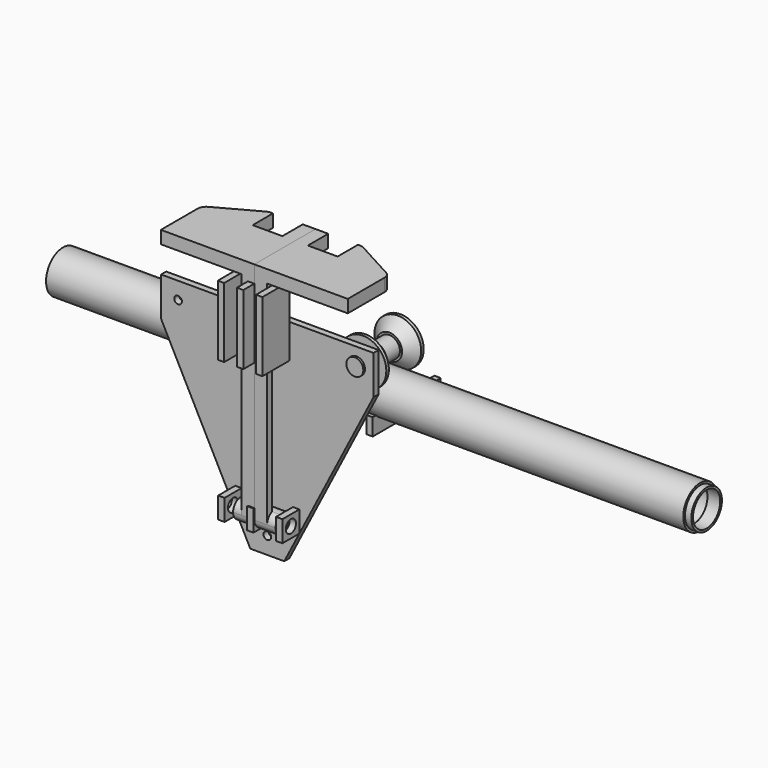
from build123d import *

# Parameters (mm, degrees)
F0_R      = 50
F0_R_2    = 45
F1_DEPTH  = 750
F2_W      = 35
F2_H      = 2.5
F6_SIZE   = 0.5
F8_DEPTH  = 15
F9_R      = 15.5
F9_R_2    = 12
F9_R_3    = 9.5
F9_R_4    = 9
F10_DEPTH = 3
F11_R     = 9
F11_R_2   = 15.5
F12_DEPTH = 15
F16_W     = 10
F16_H     = 50
F17_DEPTH = 50
F18_R     = 50
F19_DEPTH = 545.001
F21_R     = 2.5
F22_DEPTH = 12.5
F23_DEPTH = 15
F24_W     = 15
F24_H     = 50
F25_DEPTH = 50
F26_R     = 15
F27_DEPTH = 615.4994894868
F28_R     = 15
F29_DEPTH = 50
F28_W     = 15
F28_H     = 475
F30_DEPTH = 30
F31_DEPTH = 220
F32_W     = 70
F32_H     = 60
F33_DEPTH = 624.001
F34_DEPTH = 50
F35_DEPTH = 30
F36_DEPTH = 220
F37_DEPTH = 624.001
F38_R     = 45
F38_R_2   = 40
F39_DEPTH = 15
F40_W     = 15
F40_H     = 80
F40_H_2   = 84
F41_DEPTH = 80


with BuildPart() as f1:
    # F0 (on Right) → F1 (new body, symmetric)
    with BuildSketch(Plane.YZ):
        Circle(F0_R)
        Circle(F0_R_2, mode=Mode.SUBTRACT)
    extrude(amount=F1_DEPTH, both=True)

    # F38 (on face) → F39 (join, symmetric)
    with BuildSketch(Plane.YZ.offset(750)):
        Circle(F38_R)
        Circle(F38_R_2, mode=Mode.SUBTRACT)
    extrude(amount=F39_DEPTH, both=True)


with BuildPart() as f3:
    # F2 (on Right) → F3 (revolve)
    with BuildSketch(Plane.YZ):
        with Locations((0, 66.9606781187)):
            Rectangle(F2_W, F2_H)
        Polygon((-17.5, 65.7106781187), (-55, 65.7106781187), (-55, 23.2106781187), (-47.5, 23.2106781187), (-22.5, 48.2106781187), (-22.5, 53.2106781187), (22.5, 53.2106781187), (22.5, 48.2106781187), (47.5, 23.2106781187), (55, 23.2106781187), (55, 65.7106781187), (17.5, 65.7106781187), align=None)
    revolve(axis=Axis((0, 60.7904960771, 78.2106781187), (0, 1, 0)))


with BuildPart() as f5:
    # F4 (on face) → F5 (revolve)
    with BuildSketch(Plane.YZ):
        Polygon((-56, 65.7106781187), (-55, 65.7106781187), (-17.5, 65.7106781187), (-17.5, 68.2106781187), (-17.5, 69.2106781187), (-56, 69.2106781187), align=None)
    revolve(axis=Axis((0, 60.7904960771, 78.2106781187), (0, 1, 0)))

    # F6
    f6_edges = [f5.edges().sort_by_distance(p)[0] for p in [
        (0, -56, 87.210678),
        (0, -17.5, 87.210678),
        (0, -17.5, 90.710678),
        (0, -56, 90.710678),
    ]]
    chamfer(f6_edges, length=F6_SIZE)


with BuildPart() as f8:
    # F7 (on Right) → F8 (new body)
    with BuildSketch(Plane.YZ):
        with BuildLine():
            ThreePointArc((35.7071421427, -35), (0, -50), (-35.7071421427, -35))
            Line((-35.7071421427, -35), (-45, -35))
            Line((-45, -35), (-45, -75))
            Line((-45, -75), (155, -75))
            Line((155, -75), (155, -35))
            Line((155, -35), (35.7071421427, -35))
        make_face()
    extrude(amount=F8_DEPTH)


with BuildPart() as f10:
    # F9 (on face) → F10 (new body)
    with BuildSketch(Plane.XZ.offset(56)):
        with Locations((0, 78.2106781187)):
            Circle(F9_R)
        with Locations((0, 78.2106781187)):
            Circle(F9_R_2, mode=Mode.SUBTRACT)
        with Locations((0, 78.2106781187)):
            Circle(F9_R_2)
        with Locations((0, 78.2106781187)):
            Circle(F9_R_3, mode=Mode.SUBTRACT)
        with Locations((0, 78.2106781187)):
            Circle(F9_R_3)
        with Locations((0, 78.2106781187)):
            Circle(F9_R_4, mode=Mode.SUBTRACT)
    extrude(amount=F10_DEPTH)


with BuildPart() as f12:
    # F11 (on face) → F12 (new body)
    with BuildSketch(Plane.XZ.offset(59)):
        Polygon((40, 118.2106781187), (-460, 118.2106781187), (-460, 26.3970603982), (-250, -381.7893218813), (-170, -381.7893218813), (40, 26.3970603982), align=None)
        with Locations((-210, -341.7893218813)):
            Circle(F11_R, mode=Mode.SUBTRACT)
        with Locations((-420, 78.2106781187)):
            Circle(F11_R, mode=Mode.SUBTRACT)
        with Locations((-210, -78.2106781187)):
            Circle(F11_R, mode=Mode.SUBTRACT)
        with Locations((0, 78.2106781187)):
            Circle(F11_R_2, mode=Mode.SUBTRACT)
        with Locations((0, 78.2106781187)):
            Circle(F11_R_2)
        with Locations((0, 78.2106781187)):
            Circle(F11_R, mode=Mode.SUBTRACT)
    extrude(amount=F12_DEPTH)

    # F16 (on face) → F17 (join)
    with BuildSketch(Plane(origin=(0, -59, 0), x_dir=(-1, 0, 0), z_dir=(0, 1, 0))):
        with Locations((210, 0)):
            Rectangle(F16_W, F16_H)
        with Locations((210, -263.5786437627)):
            Rectangle(F16_W, F16_H)
    extrude(amount=F17_DEPTH)

    # F18 (on face) → F19 (cut, through all)
    with BuildSketch(Plane.YZ.offset(-205)):
        with Locations((0, -263.5786437627)):
            Circle(F18_R)
        with BuildLine():
            ThreePointArc((-43.3012701892, -25), (12.9409522551, -48.2962913145), (50, 0))
            ThreePointArc((50, 0), (12.9409522551, 48.2962913145), (-43.3012701892, 25))
            Line((-43.3012701892, 25), (-9, 25))
            Line((-9, 25), (-9, -25))
            Line((-9, -25), (-43.3012701892, -25))
        make_face()
        with BuildLine():
            Line((-9, 25), (-43.3012701892, 25))
            ThreePointArc((-43.3012701892, 25), (-50, 0), (-43.3012701892, -25))
            Line((-43.3012701892, -25), (-9, -25))
            Line((-9, -25), (-9, 25))
        make_face()
    extrude(amount=-F19_DEPTH, mode=Mode.SUBTRACT)

    # F24 (on face) → F25 (join)
    with BuildSketch(Plane.XZ.offset(74)):
        with Locations((-142.0015105132, -287.7893218813)):
            Rectangle(F24_W, F24_H)
        with Locations((-277.9984894868, -287.7893218813)):
            Rectangle(F24_W, F24_H)
        with Locations((-210, -287.7893218813)):
            Rectangle(F24_W, F24_H)
    extrude(amount=F25_DEPTH)

    # F26 (on face) → F27 (cut, through all)
    with BuildSketch(Plane.YZ.offset(-134.5015105132)):
        with Locations((-99, -287.7893218813)):
            Circle(F26_R)
    extrude(amount=-F27_DEPTH, mode=Mode.SUBTRACT)

    # F40 (on face) → F41 (join)
    with BuildSketch(Plane.XZ.offset(74)):
        with Locations((-255, 78.2106781187)):
            Rectangle(F40_W, F40_H)
        with Locations((-210, 78.2106781187)):
            Rectangle(F40_W, F40_H)
        with Locations((-165, 78.2106781187)):
            Rectangle(F40_W, F40_H)
        with Locations((-255, 160.2106781187)):
            Rectangle(F40_W, F40_H_2)
        with Locations((-210, 160.2106781187)):
            Rectangle(F40_W, F40_H_2)
        with Locations((-165, 160.2106781187)):
            Rectangle(F40_W, F40_H_2)
    extrude(amount=F41_DEPTH)


with BuildPart() as f15:
    # F14 (on Right) → F15 (revolve)
    with BuildSketch(Plane.YZ):
        Polygon((-74, 58.2106781187), (-74, 69.2106781187), (-74, 78.2106781187), (-79, 78.2106781187), (-79, 58.2106781187), align=None)
        Polygon((-74, 69.2106781187), (-56, 69.2106781187), (-17.5, 69.2106781187), (75, 69.2106781187), (75, 78.2106781187), (0, 78.2106781187), (-74, 78.2106781187), align=None)
    revolve(axis=Axis((0, 60.7904960771, 78.2106781187), (0, 1, 0)))

    # F21 (on face) → F22 (cut, symmetric)
    with BuildSketch(Plane(origin=(0, 0, 78.2106781187), x_dir=(1, 0, 0), z_dir=(0, 0, -1))):
        with Locations((0, -61.5)):
            Circle(F21_R)
    extrude(amount=F22_DEPTH, both=True, mode=Mode.SUBTRACT)


with BuildPart() as f23:
    # F21 (on face) → F23 (new body, symmetric)
    with BuildSketch(Plane(origin=(0, 0, 78.2106781187), x_dir=(1, 0, 0), z_dir=(0, 0, -1))):
        with Locations((0, -61.5)):
            Circle(F21_R)
    extrude(amount=F23_DEPTH, both=True)


with BuildPart() as f29:
    # F28 (on face) → F29 (new body)
    with BuildSketch(Plane.YZ.offset(-202.5)):
        with BuildLine():
            ThreePointArc((-121.5, -287.7893218813), (-99, -310.2893218813), (-76.5, -287.7893218813))
            ThreePointArc((-76.5, -287.7893218813), (-86.0096189432, -269.4181488105), (-106.5, -266.5761184457))
            ThreePointArc((-106.5, -266.5761184457), (-117.3711730709, -274.7989408246), (-121.5, -287.7893218813))
        make_face()
        with Locations((-99, -287.7893218813)):
            Circle(F28_R, mode=Mode.SUBTRACT)
    extrude(amount=F29_DEPTH)

    # F28 (on face) → F30 (join)
    with BuildSketch(Plane.YZ.offset(-202.5)):
        with BuildLine():
            ThreePointArc((-121.5, -287.7893218813), (-117.3711730709, -274.7989408246), (-106.5, -266.5761184457))
            Line((-106.5, -266.5761184457), (-106.5, -262.7893218813))
            Line((-106.5, -262.7893218813), (-121.5, -262.7893218813))
            Line((-121.5, -262.7893218813), (-121.5, -287.7893218813))
        make_face()
        with Locations((-114, -25.2893218813)):
            Rectangle(F28_W, F28_H)
    extrude(amount=F30_DEPTH)

    # F28 (on face) → F31 (join)
    with BuildSketch(Plane.YZ.offset(-202.5)):
        Polygon((-121.5, 212.2106781187), (-106.5, 212.2106781187), (58.5, 212.2106781187), (58.5, 242.2106781187), (-121.5, 242.2106781187), align=None)
    extrude(amount=F31_DEPTH)

    # F32 (on face) → F33 (cut, through all)
    with BuildSketch(Plane.XY.offset(242.2106781187)):
        with Locations((-137.5, 28.5)):
            Rectangle(F32_W, F32_H)
        Polygon((17.5, 58.5), (-92.5, 58.5), (-88.0228376735, 56.0579114583), (7.0770426136, 4.1852494835), (17.5, -1.5), align=None)
        with BuildLine():
            Line((-92.5, 58.5), (-97.5998802871, 58.5))
            ThreePointArc((-97.5998802871, 58.5), (-92.6581310607, 57.8798636368), (-88.0228376735, 56.0579114583))
            Line((-88.0228376735, 56.0579114583), (-92.5, 58.5))
        make_face()
        with BuildLine():
            ThreePointArc((7.0770426136, 4.1852494835), (14.697977385, -3.1633733677), (17.5, -13.3726619748))
            Line((17.5, -13.3726619748), (17.5, -1.5))
            Line((17.5, -1.5), (7.0770426136, 4.1852494835))
        make_face()
    extrude(amount=-F33_DEPTH, mode=Mode.SUBTRACT)


with BuildPart() as f34:
    # F28 (on face) → F34 (new body)
    with BuildSketch(Plane.YZ.offset(-202.5)):
        with BuildLine():
            ThreePointArc((-121.5, -287.7893218813), (-99, -310.2893218813), (-76.5, -287.7893218813))
            ThreePointArc((-76.5, -287.7893218813), (-86.0096189432, -269.4181488105), (-106.5, -266.5761184457))
            ThreePointArc((-106.5, -266.5761184457), (-117.3711730709, -274.7989408246), (-121.5, -287.7893218813))
        make_face()
        with Locations((-99, -287.7893218813)):
            Circle(F28_R, mode=Mode.SUBTRACT)
    extrude(amount=-F34_DEPTH)

    # F28 (on face) → F35 (join)
    with BuildSketch(Plane.YZ.offset(-202.5)):
        with Locations((-114, -25.2893218813)):
            Rectangle(F28_W, F28_H)
        with BuildLine():
            ThreePointArc((-121.5, -287.7893218813), (-117.3711730709, -274.7989408246), (-106.5, -266.5761184457))
            Line((-106.5, -266.5761184457), (-106.5, -262.7893218813))
            Line((-106.5, -262.7893218813), (-121.5, -262.7893218813))
            Line((-121.5, -262.7893218813), (-121.5, -287.7893218813))
        make_face()
    extrude(amount=-F35_DEPTH)

    # F28 (on face) → F36 (join)
    with BuildSketch(Plane.YZ.offset(-202.5)):
        Polygon((-121.5, 212.2106781187), (-106.5, 212.2106781187), (58.5, 212.2106781187), (58.5, 242.2106781187), (-121.5, 242.2106781187), align=None)
    extrude(amount=-F36_DEPTH)

    # F32 (on face) → F37 (cut, through all)
    with BuildSketch(Plane.XY.offset(242.2106781187)):
        Polygon((-316.9771623265, 56.0579114583), (-312.5, 58.5), (-422.5, 58.5), (-422.5, -1.5), (-412.0770426136, 4.1852494835), align=None)
        with Locations((-267.5, 28.5)):
            Rectangle(F32_W, F32_H)
        with BuildLine():
            ThreePointArc((-316.9771623265, 56.0579114583), (-312.3418689393, 57.8798636368), (-307.4001197129, 58.5))
            Line((-307.4001197129, 58.5), (-312.5, 58.5))
            Line((-312.5, 58.5), (-316.9771623265, 56.0579114583))
        make_face()
        with BuildLine():
            ThreePointArc((-422.5, -13.3726619748), (-419.697977385, -3.1633733677), (-412.0770426136, 4.1852494835))
            Line((-412.0770426136, 4.1852494835), (-422.5, -1.5))
            Line((-422.5, -1.5), (-422.5, -13.3726619748))
        make_face()
    extrude(amount=-F37_DEPTH, mode=Mode.SUBTRACT)


solid = Compound([f1.part, f3.part, f5.part, f8.part, f10.part, f12.part, f15.part, f23.part, f29.part, f34.part])
